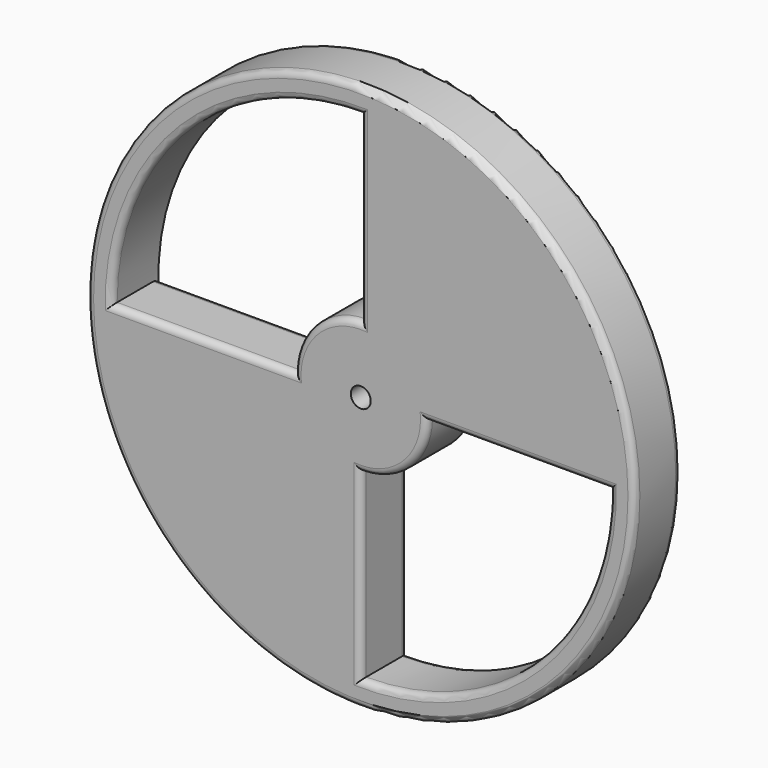
from build123d import *

# Parameters (mm, degrees)
F0_R     = 209.55
F1_DEPTH = 22.225
F3_R     = 5.08


# Not quite as in the source:
# - a feature of the source that left no trace in its solid (it failed there, or was rolled back) is left out


with BuildPart() as f1:
    # F0 (on Front) → F1 (new body, symmetric)
    with BuildSketch(Plane.XZ):
        Circle(F0_R)
        with BuildLine():
            ThreePointArc((0, 190.5), (134.703841816, 134.703841816), (190.5, 0))
            ThreePointArc((190.5, 0), (134.703841816, -134.703841816), (0, -190.5))
            ThreePointArc((0, -190.5), (-134.703841816, -134.703841816), (-190.5, 0))
            ThreePointArc((-190.5, 0), (-134.703841816, 134.703841816), (0, 190.5))
        make_face(mode=Mode.SUBTRACT)
        with BuildLine():
            ThreePointArc((0, -50.8), (35.9210244843, -35.9210244843), (50.8, 0))
            ThreePointArc((50.8, 0), (35.9210244843, 35.9210244843), (0, 50.8))
            ThreePointArc((0, 50.8), (-35.9210244843, 35.9210244843), (-50.8, 0))
            ThreePointArc((-50.8, 0), (-35.9210244843, -35.9210244843), (0, -50.8))
        make_face()
        with BuildLine():
            ThreePointArc((0, 7.62), (5.3881536726, 5.3881536726), (7.62, 0))
            ThreePointArc((7.62, 0), (-5.3881536726, -5.3881536726), (0, 7.62))
        make_face(mode=Mode.SUBTRACT)
        with BuildLine():
            Line((0, -190.5), (0, -50.8))
            ThreePointArc((0, -50.8), (-35.9210244843, -35.9210244843), (-50.8, 0))
            Line((-50.8, 0), (-190.5, 0))
            ThreePointArc((-190.5, 0), (-134.703841816, -134.703841816), (0, -190.5))
        make_face()
        with BuildLine():
            ThreePointArc((0, 50.8), (35.9210244843, 35.9210244843), (50.8, 0))
            Line((50.8, 0), (190.5, 0))
            ThreePointArc((190.5, 0), (134.703841816, 134.703841816), (0, 190.5))
            Line((0, 190.5), (0, 50.8))
        make_face()
    extrude(amount=F1_DEPTH, both=True)

    # F3
    f3_edges = [f1.edges().sort_by_distance(p)[0] for p in [
        (0, -22.225, -120.65),
        (0, 22.225, -120.65),
        (120.65, -22.225, 0),
        (-120.65, -22.225, 0),
        (0, -22.225, 120.65),
        (-209.55, 22.225, 0),
        (-209.55, -22.225, 0),
        (-134.703842, -22.225, 134.703842),
        (-35.921024, -22.225, 35.921024),
        (134.703842, -22.225, -134.703842),
        (35.921024, -22.225, -35.921024),
        (120.65, 22.225, 0),
        (134.703842, 22.225, -134.703842),
        (-120.65, 22.225, 0),
        (-35.921024, 22.225, 35.921024),
        (0, 22.225, 120.65),
    ]]
    fillet(f3_edges, radius=F3_R)


solid = f1.part
